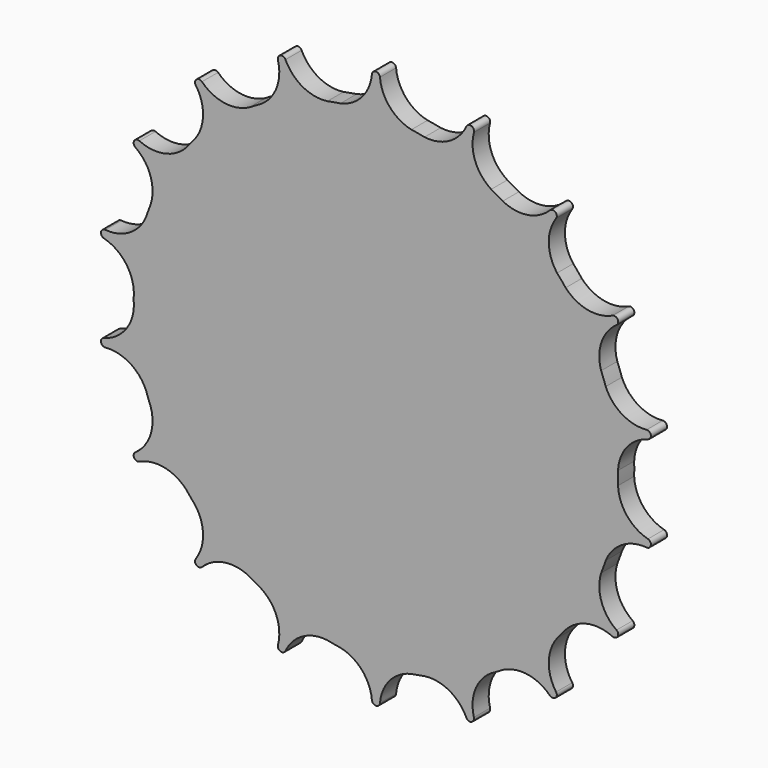
from build123d import *

# Parameters (mm, degrees)
F0_R            = 300
F1_DEPTH        = 25
F3_DEPTH        = 25
F3_COPIES_COUNT = 18


# Not quite as in the source:
# - a pattern or mirror of a feature is missing from the dataset's text; its kind, count and spacing are read off the source's solid


with BuildPart() as f1:
    # F0 (on Front) → F1 (new body)
    with BuildSketch(Plane.XZ):
        Circle(F0_R)
    extrude(amount=F1_DEPTH)

    # F2 (on face) → F3 (join, through all)
    with BuildSketch(Plane.XZ.offset(25)):
        with BuildLine():
            ThreePointArc((43.9549568499, 296.7624669131), (46.962798618, 296.1906436564), (50, 295.803989155))
            ThreePointArc((50, 295.803989155), (46.9799228296, 296.2986446998), (43.9549568499, 296.7624669131))
        make_face()
        with BuildLine():
            ThreePointArc((-50, 295.803989155), (-46.962798618, 296.1906436564), (-43.9549568499, 296.7624669131))
            ThreePointArc((-43.9549568499, 296.7624669131), (-46.9799228296, 296.2986446998), (-50, 295.803989155))
        make_face()
        with BuildLine():
            ThreePointArc((-43.9549568499, 296.7624669131), (0, 300), (43.9549568499, 296.7624669131))
            ThreePointArc((43.9549568499, 296.7624669131), (17.1882851118, 312.6207310432), (4.9811623415, 341.2376038778))
            ThreePointArc((4.9811623415, 341.2376038778), (0, 345.803989155), (-4.9811623415, 341.2376038778))
            ThreePointArc((-4.9811623415, 341.2376038778), (-17.1882851118, 312.6207310432), (-43.9549568499, 296.7624669131))
        make_face()
    f3 = extrude(amount=-F3_DEPTH)

    # F3_copies: F3 ×18 about axis
    f3_copies_axis = Axis((0, 0, 0), (0, 1, 0))
    for i in range(1, F3_COPIES_COUNT):
        add(f3.rotate(f3_copies_axis, i * 360 / F3_COPIES_COUNT))


solid = f1.part
